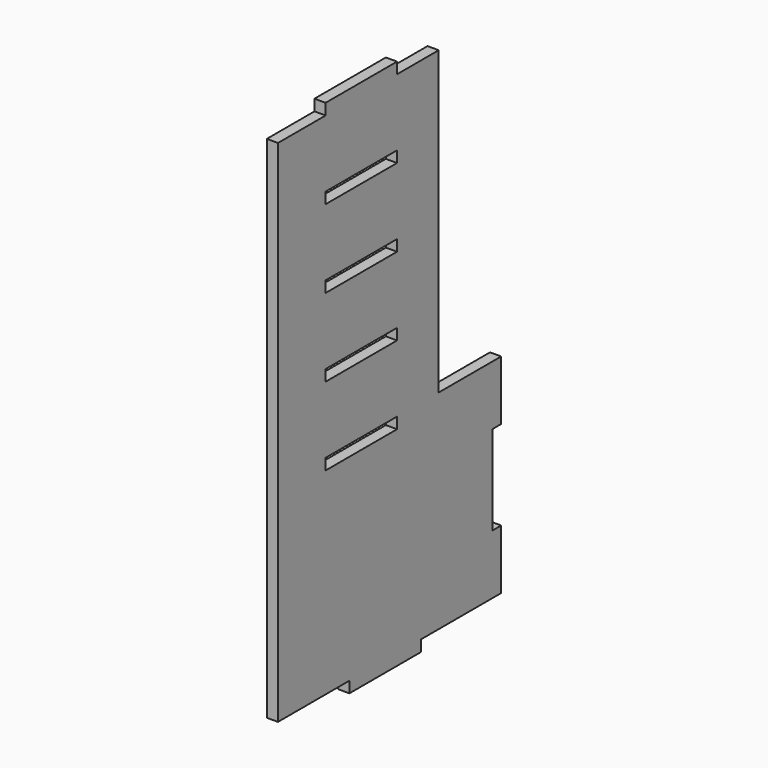
from build123d import *

# Parameters (mm, degrees)
F0_W     = 152.4
F0_H     = 19.05
F1_DEPTH = 19.05


# Not quite as in the source:
# - a feature names something its author has since deleted; it is built from what else it names


with BuildPart() as f1:
    # F0 (on Right) → F1 (new body)
    with BuildSketch(Plane.YZ):
        Polygon((-69.85, 0), (-171.45, 0), (-171.45, -869.95), (-19.05, -869.95), (40.3552334547, -869.95), (133.35, -869.95), (171.45, -869.95), (171.45, -514.35), (171.45, 0), (82.55, 0), align=None)
        with Locations((6.35, -523.875)):
            Rectangle(F0_W, F0_H, mode=Mode.SUBTRACT)
        with Locations((6.35, -390.525)):
            Rectangle(F0_W, F0_H, mode=Mode.SUBTRACT)
        with Locations((6.35, -257.175)):
            Rectangle(F0_W, F0_H, mode=Mode.SUBTRACT)
        with Locations((6.35, -123.825)):
            Rectangle(F0_W, F0_H, mode=Mode.SUBTRACT)
        Polygon((40.3552334547, -869.95), (-19.05, -869.95), (-19.05, -889), (133.35, -889), (133.35, -869.95), align=None)
        Polygon((304.8, -514.35), (171.45, -514.35), (171.45, -869.95), (304.8, -869.95), (304.8, -768.35), (285.75, -768.35), (285.75, -615.95), (304.8, -615.95), align=None)
        with Locations((6.35, 9.525)):
            Rectangle(F0_W, F0_H)
    extrude(amount=F1_DEPTH)


solid = f1.part
